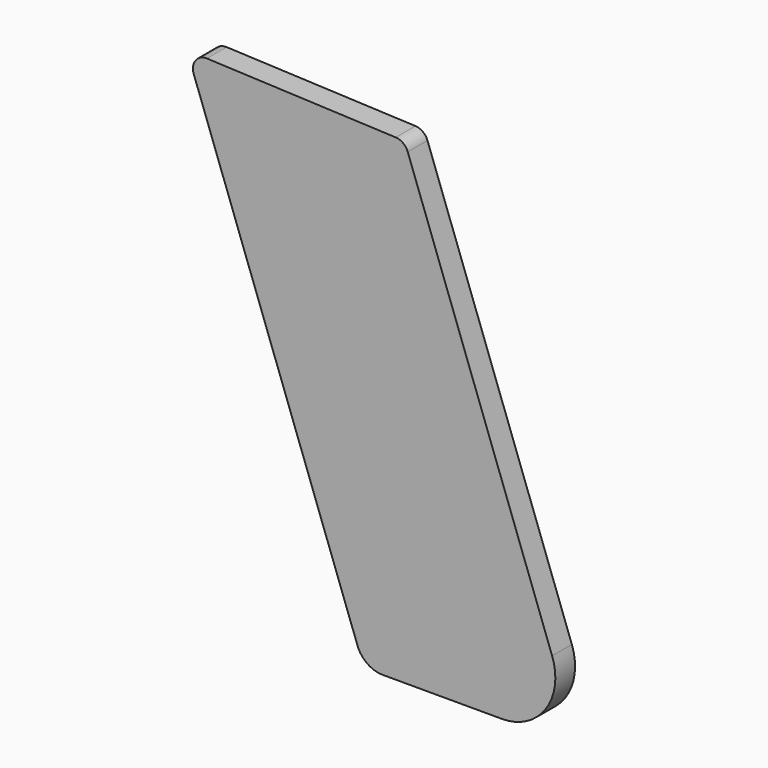
from build123d import *

# Parameters (mm, degrees)
F1_DEPTH = 5.842
F2_R     = 6.35
F3_R     = 12.7
F6_DEPTH = 25.4
F7_R     = 3.175


# Not quite as in the source:
# - a length typed as a fraction of an inch, garbled in the dataset ("3 / 203.2 mm" for 3/8 in), is restored


with BuildPart() as f1:
    # F0 (on Front) → F1 (new body)
    with BuildSketch(Plane.XZ):
        Polygon((50.8, 0), (0, 0), (55.4690637022, -152.4), (106.2690637022, -152.4), align=None)
    extrude(amount=F1_DEPTH)

    # F2
    f2_edges = [f1.edges().sort_by_distance(p)[0] for p in [
        (55.469064, -2.921, -152.4),
        (50.8, -2.921, 0),
        (0, -2.921, 0),
    ]]
    fillet(f2_edges, radius=F2_R)

    # F3
    f3_edges = [f1.edges().sort_by_distance(p)[0] for p in [
        (106.269064, -2.921, -152.4),
    ]]
    fillet(f3_edges, radius=F3_R)

    # F5 (on face) → F6 (cut)
    with BuildSketch(Plane.XZ.offset(5.842)):
        Polygon((109.8922565579, 0), (-38.8115942478, 0), (-38.8115942478, -34.925), (109.8922565579, -41.275), align=None)
    extrude(amount=-F6_DEPTH, mode=Mode.SUBTRACT)

    # F7
    f7_edges = [f1.edges().sort_by_distance(p)[0] for p in [
        (65.127115, -2.921, -39.363424),
        (13.525097, -2.921, -37.159898),
    ]]
    fillet(f7_edges, radius=F7_R)


solid = f1.part
